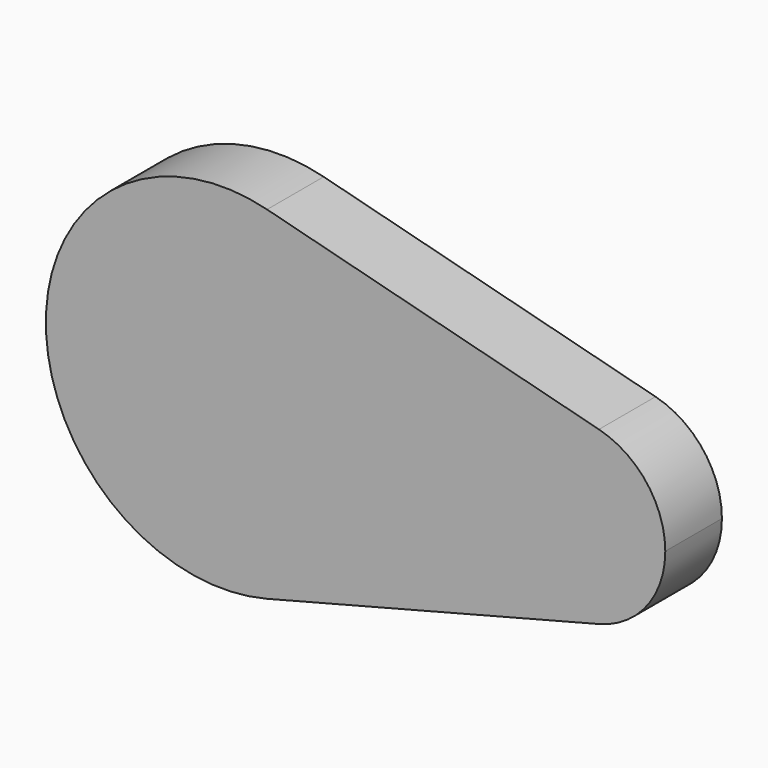
from build123d import *

# Parameters (mm, degrees)
F1_DEPTH = 10


# Not quite as in the source:
# - the program builds the solid bodies; features that only make, move or delete a surface that nothing else refers to are left out


with BuildPart() as f1:
    # F0 (on Front) → F1 (new body)
    with BuildSketch(Plane.XZ):
        with BuildLine():
            ThreePointArc((-8.1000001146, 0), (-13.3357647385, 15.3093108924), (-26.8500001146, 24.2061459138))
            ThreePointArc((-26.8500001146, 24.2061459138), (-58.1000001146, 0), (-26.8500001146, -24.2061459138))
            ThreePointArc((-26.8500001146, -24.2061459138), (-13.3357647385, -15.3093108924), (-8.1000001146, 0))
        make_face()
        with BuildLine():
            Line((20.0249998854, 12.1030729569), (-26.8500001146, 24.2061459138))
            ThreePointArc((-26.8500001146, 24.2061459138), (-13.3357647385, 15.3093108924), (-8.1000001146, 0))
            ThreePointArc((-8.1000001146, 0), (-13.3357647385, -15.3093108924), (-26.8500001146, -24.2061459138))
            Line((-26.8500001146, -24.2061459138), (20.0249998854, -12.1030729569))
            ThreePointArc((20.0249998854, -12.1030729569), (4.3999998854, 0), (20.0249998854, 12.1030729569))
        make_face()
        with BuildLine():
            ThreePointArc((29.3999998854, 0), (26.7821175735, 7.6546554462), (20.0249998854, 12.1030729569))
            ThreePointArc((20.0249998854, 12.1030729569), (4.3999998854, 0), (20.0249998854, -12.1030729569))
            ThreePointArc((20.0249998854, -12.1030729569), (26.7821175735, -7.6546554462), (29.3999998854, 0))
        make_face()
    extrude(amount=F1_DEPTH)


solid = f1.part
